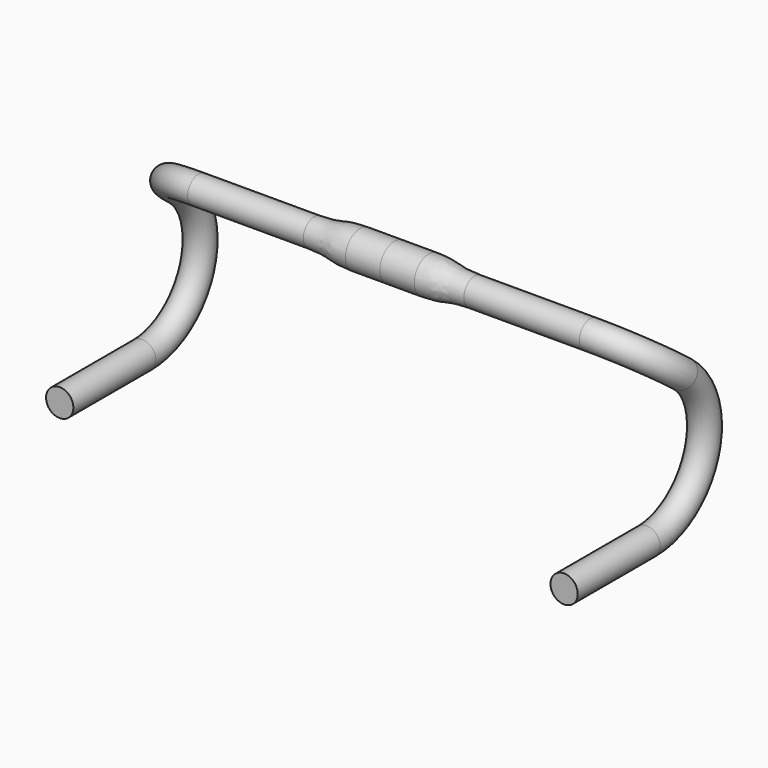
from build123d import *

# Parameters (mm, degrees)
F4_R       = 11.90625
F11_FACE_R = 11.90625
F13_FACE_R = 11.90625


with BuildPart() as f11:
    # F11: sweep along a path in F8, F10
    with BuildLine(Plane(origin=(220, 0, 0), x_dir=(0, -1, 0), z_dir=(-1, 0, 0))) as f11_path:
        Line((90, -143.09375), (0, -143.09375))
        ThreePointArc((0, -143.09375), (-59.6673406444, -100.5092600912), (-38.7909423113, -30.2397338867))
    with BuildLine(Plane(origin=(0, 0, 0), x_dir=(1, 0, 0), z_dir=(0, 0.6148143407, 0.788671875))) as f11_path_2:
        ThreePointArc((170.8148527405, 0), (205.5940039014, 14.4059960986), (220, 49.1851472595))
    # F4 (on line) → F11 (sweep)
    with BuildSketch(Plane(origin=(0, -90, 0), x_dir=(-1, 0, 0), z_dir=(0, 1, 0))):
        with Locations((-220, -143.09375)):
            Circle(F4_R)
    sweep(path=f11_path.line + f11_path_2.line)



with BuildPart() as f13:
    # F12 (on 3pt) → F13 (revolve)
    with BuildSketch(Plane(origin=(0, 0, 0), x_dir=(1, 0, 0), z_dir=(0, 0.6148143407, 0.788671875))):
        with BuildLine():
            Line((0, 0), (0, -15.9))
            Line((0, -15.9), (30, -15.9))
            add(Edge.make_bspline(
                [(70, -11.90625), (50, -11.90625), (50, -15.9), (30, -15.9)],
                knots=[0, 0, 0, 0, 40.1988810673, 40.1988810673, 40.1988810673, 40.1988810673], degree=3))
            Line((70, -11.90625), (70, 0))
            Line((70, 0), (0, 0))
        make_face()
    revolve(axis=Axis((85.4074263703, 0, 0), (-1, 0, 0)))


with BuildPart() as f11_1:
    add(f11.part)

    add(f13.part)  # F14 merges F13
    # F11_face (on face) → F14 section 0
    with BuildSketch(Plane(origin=(170.8148527405, 0, 0), x_dir=(0, -1, 0), z_dir=(-1, 0, 0))):
        Circle(F11_FACE_R)
    # F13_face (on face) → F14 section 1
    with BuildSketch(Plane.YZ.offset(70)):
        Circle(F13_FACE_R)
    loft()

    # F15: F11 across plane


with BuildPart() as f11_2:
    add(f11_1.part)
    add(f11_1.part.mirror(Plane.YZ))


solid = f11_2.part
